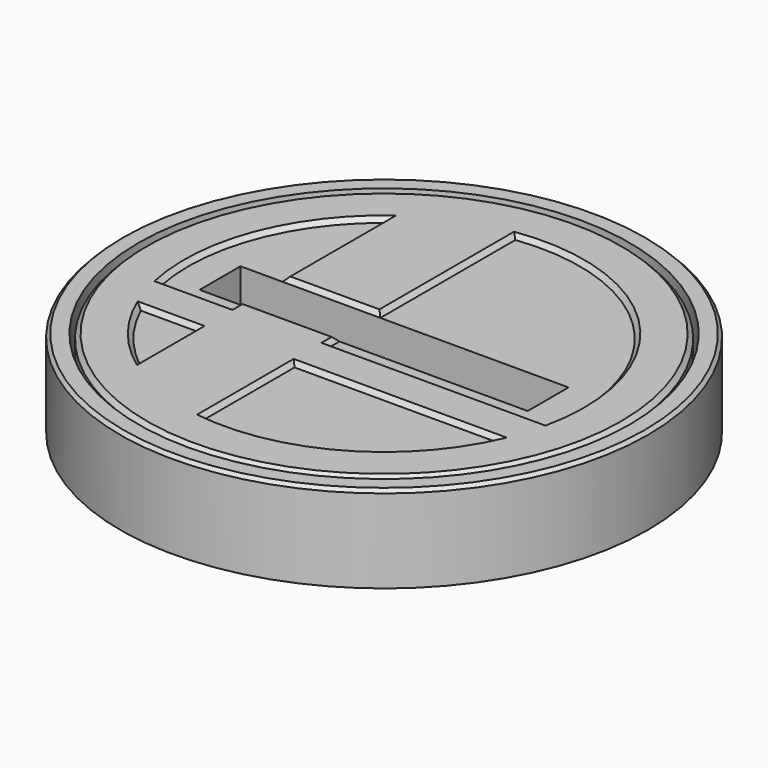
from build123d import *

# Parameters (mm, degrees)
F0_R     = 22.225
F1_DEPTH = 8
F2_DEPTH = 0.4
F3_W     = 30.2
F3_H     = 4.7
F4_DEPTH = 5.3
F5_SIZE  = 0.39999
F6_R     = 24.3
F6_R_2   = 22.625
F7_DEPTH = 8
F8_SIZE  = 0.3


# Not quite as in the source:
# - a fillet or chamfer is up to 0.001 mm smaller than in the source, because OpenCascade refuses the exact size


with BuildPart() as f1:
    # F0 (on Top) → F1 (new body)
    with BuildSketch(Plane.XY):
        Circle(F0_R)
        with BuildLine():
            ThreePointArc((-11.225, -14.1031911283), (-14.1885435786, -11.1169175637), (-16.3791025395, -7.525))
            Line((-16.3791025395, -7.525), (-11.225, -7.525))
            Line((-11.225, -7.525), (-11.225, -14.1031911283))
        make_face(mode=Mode.SUBTRACT)
        with BuildLine():
            Line((-2.225, -17.8871462229), (-2.225, -7.525))
            Line((-2.225, -7.525), (16.3791025395, -7.525))
            ThreePointArc((16.3791025395, -7.525), (8.7708707242, -15.7471410656), (-2.225, -17.8871462229))
        make_face(mode=Mode.SUBTRACT)
        with BuildLine():
            ThreePointArc((-17.6769624087, -3.525), (-16.9268762145, 6.1952793817), (-11.225, 14.1031911283))
            Line((-11.225, 14.1031911283), (-11.225, -3.525))
            Line((-11.225, -3.525), (-17.6769624087, -3.525))
        make_face(mode=Mode.SUBTRACT)
        with BuildLine():
            Line((-2.225, -3.525), (-2.225, 17.8871462229))
            ThreePointArc((-2.225, 17.8871462229), (13.2026810549, 12.2715051221), (17.6769624087, -3.525))
            Line((17.6769624087, -3.525), (-2.225, -3.525))
        make_face(mode=Mode.SUBTRACT)
        with BuildLine():
            Line((-11.225, -7.525), (-16.3791025395, -7.525))
            ThreePointArc((-16.3791025395, -7.525), (-14.1885435786, -11.1169175637), (-11.225, -14.1031911283))
            Line((-11.225, -14.1031911283), (-11.225, -7.525))
        make_face()
        with BuildLine():
            Line((-11.225, -3.525), (-11.225, 14.1031911283))
            ThreePointArc((-11.225, 14.1031911283), (-16.9268762145, 6.1952793817), (-17.6769624087, -3.525))
            Line((-17.6769624087, -3.525), (-11.225, -3.525))
        make_face()
        with BuildLine():
            ThreePointArc((17.6769624087, -3.525), (13.2026810549, 12.2715051221), (-2.225, 17.8871462229))
            Line((-2.225, 17.8871462229), (-2.225, -3.525))
            Line((-2.225, -3.525), (17.6769624087, -3.525))
        make_face()
        with BuildLine():
            Line((16.3791025395, -7.525), (-2.225, -7.525))
            Line((-2.225, -7.525), (-2.225, -17.8871462229))
            ThreePointArc((-2.225, -17.8871462229), (8.7708707242, -15.7471410656), (16.3791025395, -7.525))
        make_face()
    extrude(amount=-F1_DEPTH)

    # F0 (on Top) → F2 (cut)
    with BuildSketch(Plane.XY):
        with BuildLine():
            Line((-11.225, -3.525), (-11.225, 14.1031911283))
            ThreePointArc((-11.225, 14.1031911283), (-16.9268762145, 6.1952793817), (-17.6769624087, -3.525))
            Line((-17.6769624087, -3.525), (-11.225, -3.525))
        make_face()
        with BuildLine():
            ThreePointArc((17.6769624087, -3.525), (13.2026810549, 12.2715051221), (-2.225, 17.8871462229))
            Line((-2.225, 17.8871462229), (-2.225, -3.525))
            Line((-2.225, -3.525), (17.6769624087, -3.525))
        make_face()
        with BuildLine():
            Line((16.3791025395, -7.525), (-2.225, -7.525))
            Line((-2.225, -7.525), (-2.225, -17.8871462229))
            ThreePointArc((-2.225, -17.8871462229), (8.7708707242, -15.7471410656), (16.3791025395, -7.525))
        make_face()
        with BuildLine():
            Line((-11.225, -7.525), (-16.3791025395, -7.525))
            ThreePointArc((-16.3791025395, -7.525), (-14.1885435786, -11.1169175637), (-11.225, -14.1031911283))
            Line((-11.225, -14.1031911283), (-11.225, -7.525))
        make_face()
    extrude(amount=-F2_DEPTH, mode=Mode.SUBTRACT)

    # F3 (on Top) → F4 (cut)
    with BuildSketch(Plane.XY):
        Rectangle(F3_W, F3_H)
    extrude(amount=-F4_DEPTH, mode=Mode.SUBTRACT)

    # F5 (size 0.4 in the source; OpenCascade refuses exactly that, so slightly less here)
    f5_edges = [f1.edges().sort_by_distance(p)[0] for p in [
        (-11.225, 8.226596, 0),
        (-16.926876, 6.195279, 0),
        (-14.450981, -3.525, 0),
        (-11.225, -2.9375, 0),
        (13.202681, 12.271505, 0),
        (-2.225, 10.118573, 0),
        (7.725981, -3.525, 0),
        (7.077051, -7.525, 0),
        (8.770871, -15.747141, 0),
        (-2.225, -2.9375, 0),
        (-2.225, -12.706073, 0),
        (-13.802051, -7.525, 0),
        (-14.188544, -11.116918, 0),
        (-11.225, -10.814096, 0),
        (-6.725, 2.35, 0),
        (-6.725, -2.35, 0),
        (-22.225, 0, 0),
    ]]
    chamfer(f5_edges, length=F5_SIZE)


with BuildPart() as f7:
    # F6 (on Top) → F7 (new body, through all)
    with BuildSketch(Plane.XY):
        Circle(F6_R)
        Circle(F6_R_2, mode=Mode.SUBTRACT)
    extrude(amount=-F7_DEPTH)

    # F8
    f8_edges = [f7.edges().sort_by_distance(p)[0] for p in [
        (-24.3, 0, 0),
    ]]
    chamfer(f8_edges, length=F8_SIZE)


solid = Compound([f1.part, f7.part])
